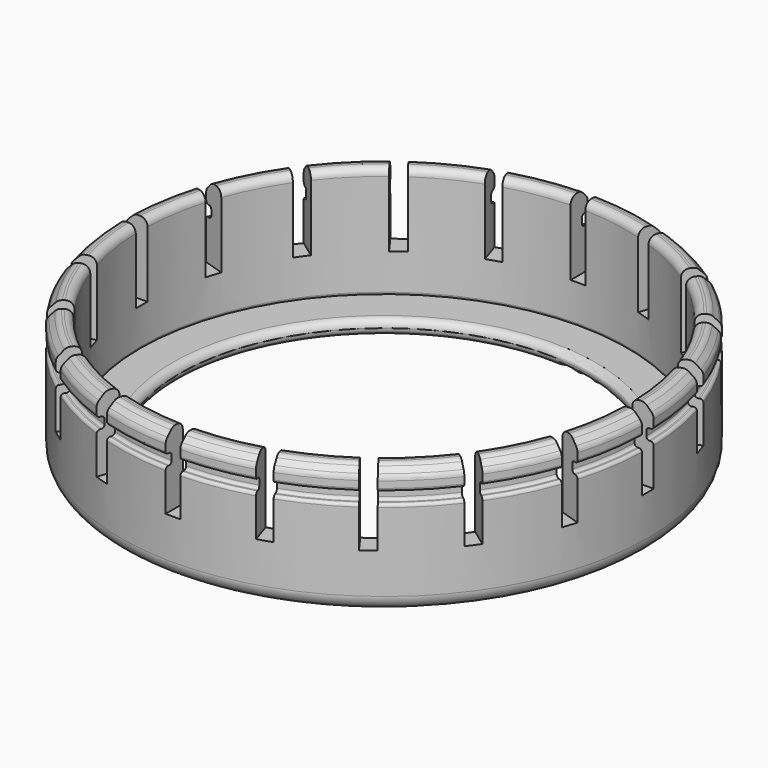
from build123d import *

# Parameters (mm, degrees)
F2_W            = 2.54
F2_H            = 3.7276002762
F3_DEPTH        = 12.7
F3_COPIES_COUNT = 20
F4_R            = 0.508
F5_R            = 1.26999
F6_R            = 2.54


# Not quite as in the source:
# - a fillet or chamfer is up to 0.001 mm smaller than in the source, because OpenCascade refuses the exact size
# - a pattern or mirror of a feature is missing from the dataset's text; its kind, count and spacing are read off the source's solid


with BuildPart() as f1:
    # F0 (on Front) → F1 (revolve)
    with BuildSketch(Plane.XZ):
        Polygon((35.3695, 2.54), (35.3695, 0), (45.72, 0), (45.72, 16.6116), (44.45, 16.6116), (44.45, 18.5166), (45.72, 18.5166), (45.72, 20.6889304253), (44.1839304253, 22.225), (42.0116, 22.225), (42.0116, 2.794), (43.8658, 2.794), (43.8658, 2.54), align=None)
    revolve(axis=Axis((0, 0, 11.1125), (0, 0, -1)))

    # F2 (on face) → F3 (cut)
    with BuildSketch(Plane.XY.offset(22.225)):
        with Locations((0, 43.8561998619)):
            Rectangle(F2_W, F2_H)
    f3 = extrude(amount=-F3_DEPTH, mode=Mode.SUBTRACT)

    # F3_copies: F3 ×20 about axis
    f3_copies_axis = Axis((0, 0, 0), (0, 0, 1))
    for i in range(1, F3_COPIES_COUNT):
        add(f3.rotate(f3_copies_axis, i * 360 / F3_COPIES_COUNT), mode=Mode.SUBTRACT)

    # F4
    f4_edges = [f1.edges().sort_by_distance(p)[0] for p in [
        (6.953512, 43.902747, 18.5166),
        (20.179878, 39.60524, 18.5166),
        (31.430896, 31.430896, 18.5166),
        (39.60524, 20.179878, 18.5166),
        (43.902747, 6.953512, 18.5166),
        (39.60524, -20.179878, 18.5166),
        (31.430896, -31.430896, 18.5166),
        (20.179878, -39.60524, 18.5166),
        (6.953512, -43.902747, 18.5166),
        (-6.953512, -43.902747, 18.5166),
        (-20.179878, -39.60524, 18.5166),
        (-31.430896, -31.430896, 18.5166),
        (-39.60524, -20.179878, 18.5166),
        (-43.902747, -6.953512, 18.5166),
        (-43.902747, 6.953512, 18.5166),
        (-39.60524, 20.179878, 18.5166),
        (-31.430896, 31.430896, 18.5166),
        (-20.179878, 39.60524, 18.5166),
        (-6.953512, 43.902747, 18.5166),
        (43.902747, -6.953512, 18.5166),
        (6.953512, 43.902747, 16.6116),
        (20.179878, 39.60524, 16.6116),
        (31.430896, 31.430896, 16.6116),
        (39.60524, 20.179878, 16.6116),
        (43.902747, 6.953512, 16.6116),
        (39.60524, -20.179878, 16.6116),
        (31.430896, -31.430896, 16.6116),
        (20.179878, -39.60524, 16.6116),
        (6.953512, -43.902747, 16.6116),
        (-6.953512, -43.902747, 16.6116),
        (-20.179878, -39.60524, 16.6116),
        (-31.430896, -31.430896, 16.6116),
        (-39.60524, -20.179878, 16.6116),
        (-43.902747, -6.953512, 16.6116),
        (-43.902747, 6.953512, 16.6116),
        (-39.60524, 20.179878, 16.6116),
        (-31.430896, 31.430896, 16.6116),
        (-20.179878, 39.60524, 16.6116),
        (-6.953512, 43.902747, 16.6116),
        (43.902747, -6.953512, 16.6116),
        (45.157111, 7.152184, 16.6116),
        (40.736818, 20.756446, 16.6116),
        (32.328922, 32.328922, 16.6116),
        (20.756446, 40.736818, 16.6116),
        (7.152184, 45.157111, 16.6116),
        (-7.152184, 45.157111, 16.6116),
        (-20.756446, 40.736818, 16.6116),
        (-32.328922, 32.328922, 16.6116),
        (-40.736818, 20.756446, 16.6116),
        (-45.157111, 7.152184, 16.6116),
        (-45.157111, -7.152184, 16.6116),
        (-40.736818, -20.756446, 16.6116),
        (-32.328922, -32.328922, 16.6116),
        (-20.756446, -40.736818, 16.6116),
        (-7.152184, -45.157111, 16.6116),
        (7.152184, -45.157111, 16.6116),
        (20.756446, -40.736818, 16.6116),
        (32.328922, -32.328922, 16.6116),
        (40.736818, -20.756446, 16.6116),
        (45.157111, -7.152184, 16.6116),
        (7.152184, 45.157111, 18.5166),
        (20.756446, 40.736818, 18.5166),
        (32.328922, 32.328922, 18.5166),
        (40.736818, 20.756446, 18.5166),
        (45.157111, 7.152184, 18.5166),
        (40.736818, -20.756446, 18.5166),
        (32.328922, -32.328922, 18.5166),
        (20.756446, -40.736818, 18.5166),
        (7.152184, -45.157111, 18.5166),
        (-7.152184, -45.157111, 18.5166),
        (-20.756446, -40.736818, 18.5166),
        (-32.328922, -32.328922, 18.5166),
        (-40.736818, -20.756446, 18.5166),
        (-45.157111, -7.152184, 18.5166),
        (-45.157111, 7.152184, 18.5166),
        (-40.736818, 20.756446, 18.5166),
        (-32.328922, 32.328922, 18.5166),
        (-20.756446, 40.736818, 18.5166),
        (-7.152184, 45.157111, 18.5166),
        (45.157111, -7.152184, 18.5166),
        (-42.0116, 0, 2.794),
    ]]
    fillet(f4_edges, radius=F4_R)

    # F5 (radius 1.27 in the source; OpenCascade refuses exactly that, so slightly less here)
    f5_edges = [f1.edges().sort_by_distance(p)[0] for p in [
        (40.736818, -20.756446, 20.68893),
        (32.328922, -32.328922, 20.68893),
        (20.756446, -40.736818, 20.68893),
        (7.152184, -45.157111, 20.68893),
        (-7.152184, -45.157111, 20.68893),
        (-20.756446, -40.736818, 20.68893),
        (-32.328922, -32.328922, 20.68893),
        (-40.736818, -20.756446, 20.68893),
        (-45.157111, -7.152184, 20.68893),
        (-45.157111, 7.152184, 20.68893),
        (-40.736818, 20.756446, 20.68893),
        (-32.328922, 32.328922, 20.68893),
        (-20.756446, 40.736818, 20.68893),
        (-7.152184, 45.157111, 20.68893),
        (45.157111, -7.152184, 20.68893),
        (7.152184, 45.157111, 20.68893),
        (20.756446, 40.736818, 20.68893),
        (32.328922, 32.328922, 20.68893),
        (40.736818, 20.756446, 20.68893),
        (45.157111, 7.152184, 20.68893),
        (39.36817, -20.059085, 22.225),
        (31.242757, -31.242757, 22.225),
        (20.059085, -39.36817, 22.225),
        (6.91189, -43.639953, 22.225),
        (-6.91189, -43.639953, 22.225),
        (-20.059085, -39.36817, 22.225),
        (-31.242757, -31.242757, 22.225),
        (-39.36817, -20.059085, 22.225),
        (-43.639953, -6.91189, 22.225),
        (-43.639953, 6.91189, 22.225),
        (-39.36817, 20.059085, 22.225),
        (-31.242757, 31.242757, 22.225),
        (-20.059085, 39.36817, 22.225),
        (-6.91189, 43.639953, 22.225),
        (43.639953, -6.91189, 22.225),
        (6.91189, 43.639953, 22.225),
        (20.059085, 39.36817, 22.225),
        (31.242757, 31.242757, 22.225),
        (39.36817, 20.059085, 22.225),
        (43.639953, 6.91189, 22.225),
        (-35.3695, 0, 2.54),
        (-35.3695, 0, 0),
        (41.494367, 6.572062, 22.225),
        (37.43261, 19.072867, 22.225),
        (29.706687, 29.706687, 22.225),
        (19.072867, 37.43261, 22.225),
        (6.572062, 41.494367, 22.225),
        (-6.572062, 41.494367, 22.225),
        (-19.072867, 37.43261, 22.225),
        (-29.706687, 29.706687, 22.225),
        (-37.43261, 19.072867, 22.225),
        (-41.494367, 6.572062, 22.225),
        (-41.494367, -6.572062, 22.225),
        (-37.43261, -19.072867, 22.225),
        (-29.706687, -29.706687, 22.225),
        (-19.072867, -37.43261, 22.225),
        (-6.572062, -41.494367, 22.225),
        (6.572062, -41.494367, 22.225),
        (19.072867, -37.43261, 22.225),
        (29.706687, -29.706687, 22.225),
        (37.43261, -19.072867, 22.225),
        (41.494367, -6.572062, 22.225),
    ]]
    fillet(f5_edges, radius=F5_R)

    # F6
    f6_edges = [f1.edges().sort_by_distance(p)[0] for p in [
        (-45.72, 0, 0),
    ]]
    fillet(f6_edges, radius=F6_R)


solid = f1.part
